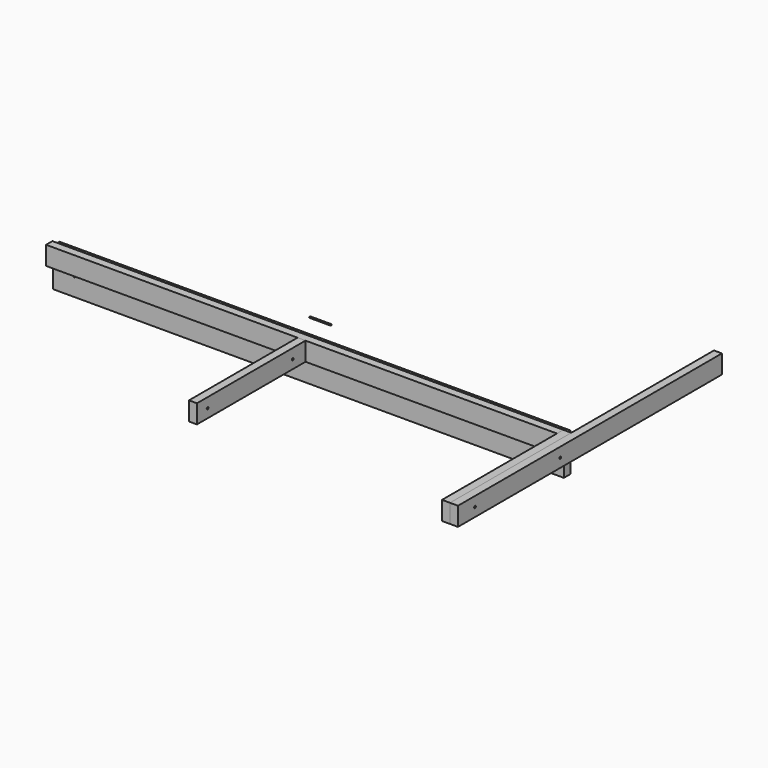
from build123d import *

# Parameters (mm, degrees)
F0_W        = 38.1
F0_H        = 184.15
F1_DEPTH    = 1219.2
F2_W        = 38.1
F2_H        = 88.9
F3_DEPTH    = 1219.2
F4_W        = 723.9
F4_H        = 88.9
F5_DEPTH    = 38.1
F6_W        = 38.1
F6_H        = 88.9
F7_DEPTH    = 647.7
F8_R        = 4.7625
F9_DEPTH    = 765.176
F11_DEPTH   = 13.49375
F12_W       = 38.1
F12_H       = 88.9
F13_DEPTH   = 1574.8
F15_D       = 10.3124
F15_DEPTH   = 1314.451
F15_2_D     = 10.3124
F15_2_DEPTH = 1314.451
F15_3_D     = 10.3124
F15_3_DEPTH = 1314.451
F16_R       = 3.175
F17_DEPTH   = 50.8
F18_R       = 1.9939
F19_DEPTH   = 50.8


with BuildPart() as f1:
    # F0 (on Right) → F1 (new body, symmetric)
    with BuildSketch(Plane.YZ):
        with Locations((-19.05, -92.075)):
            Rectangle(F0_W, F0_H)
    extrude(amount=F1_DEPTH, both=True)

    # F8 (on face) → F9 (cut, through all)
    with BuildSketch(Plane(origin=(0, 0, 0), x_dir=(-1, 0, 0), z_dir=(0, 1, 0))):
        with Locations((-1117.6, -97.63125)):
            Circle(F8_R)
        with Locations((1117.6, -97.6376)):
            Circle(F8_R)
    extrude(amount=-F9_DEPTH, mode=Mode.SUBTRACT)


with BuildPart() as f3:
    # F2 (on Right) → F3 (new body, symmetric)
    with BuildSketch(Plane.YZ):
        with Locations((-60.325, -25.4)):
            Rectangle(F2_W, F2_H)
    extrude(amount=F3_DEPTH, both=True)


with BuildPart() as f5:
    # F4 (on face) → F5 (new body)
    with BuildSketch(Plane.YZ.offset(1219.2)):
        with Locations((-403.225, -25.4)):
            Rectangle(F4_W, F4_H)
    extrude(amount=F5_DEPTH)

    # F15 (through all, one way)
    with BuildSketch(Plane.YZ.offset(1295.4)):
        with Locations((-663.575, -27.5529492646), (-155.575, -27.5529492646)):
            Circle(F15_D / 2)
    extrude(amount=-F15_DEPTH, mode=Mode.SUBTRACT)


with BuildPart() as f7:
    # F6 (on face) → F7 (new body)
    with BuildSketch(Plane.XZ.offset(79.375)):
        with Locations((0, -25.4)):
            Rectangle(F6_W, F6_H)
    extrude(amount=F7_DEPTH)

    # F15#2 (through all, one way)
    with BuildSketch(Plane.YZ.offset(1295.4)):
        with Locations((-663.575, -27.5529492646), (-155.575, -27.5529492646)):
            Circle(F15_2_D / 2)
    extrude(amount=-F15_2_DEPTH, mode=Mode.SUBTRACT)


with BuildPart() as f11:
    # F10 (on face) → F11 (new body)
    with BuildSketch(Plane(origin=(0, 0, -69.85), x_dir=(1, 0, 0), z_dir=(0, 0, -1))):
        Polygon((1219.2, 41.275), (1257.3, 41.275), (1257.3, 168.275), (1219.2, 130.175), align=None)
        Polygon((1130.3, 41.275), (1219.2, 41.275), (1219.2, 130.175), align=None)
    extrude(amount=F11_DEPTH)


with BuildPart() as f13:
    # F12 (on face) → F13 (new body)
    with BuildSketch(Plane.XZ.offset(765.175)):
        with Locations((1276.35, -25.4)):
            Rectangle(F12_W, F12_H)
    extrude(amount=-F13_DEPTH)

    # F15#3 (through all, one way)
    with BuildSketch(Plane.YZ.offset(1295.4)):
        with Locations((-663.575, -27.5529492646), (-155.575, -27.5529492646)):
            Circle(F15_3_D / 2)
    extrude(amount=-F15_3_DEPTH, mode=Mode.SUBTRACT)


with BuildPart() as f17:
    # F16 (on Right) → F17 (new body, symmetric)
    with BuildSketch(Plane.YZ):
        with Locations((33.3801843226, 49.415204674)):
            Circle(F16_R)
    extrude(amount=F17_DEPTH, both=True)


with BuildPart() as f19_tool:
    # F18 (on face) → F19 (new body, symmetric)
    with BuildSketch(Plane(origin=(0, -41.275, 0), x_dir=(-1, 0, 0), z_dir=(0, 1, 0))):
        with Locations((8.9916, -55.3466)):
            Circle(F18_R)
        with Locations((-8.9916, -55.3466)):
            Circle(F18_R)
    extrude(amount=F19_DEPTH, both=True)


with BuildPart() as f1_1:
    add(f1.part)

    # F19: cut by f19_tool
    add(f19_tool.part, mode=Mode.SUBTRACT)


with BuildPart() as f3_1:
    add(f3.part)

    # F19: cut by f19_tool
    add(f19_tool.part, mode=Mode.SUBTRACT)


solid = Compound([f5.part, f7.part, f11.part, f13.part, f17.part, f1_1.part, f3_1.part])
